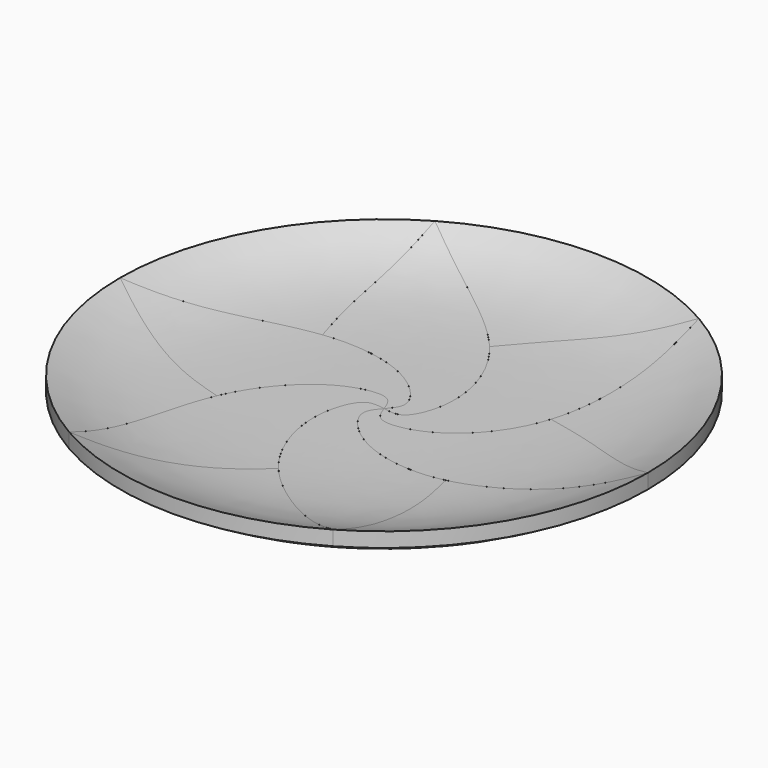
from build123d import *

# Parameters (mm, degrees)
F1_DEPTH  = 25.4
F2_ANGLE  = 60
F3_ANGLE  = 60
F4_ANGLE  = 180
F6_DEPTH  = 25.4
F10_R     = 127
F11_DEPTH = 25.4


# Not quite as in the source:
# - after a boolean that leaves OpenCascade's solid faulty, fix() repairs it


with BuildPart() as f1:
    # F0 (on Top) → F1 (new body)
    with BuildSketch(Plane.XY):
        with BuildLine():
            add(Edge.make_bspline(
                [(57.15, 98.9867036526), (42.865067123, 90.4469959657), (18.1027123706, 75.6437572636), (5.3822632476, 62.6485279549), (0, 57.15)],
                knots=[0, 0, 0, 0, 0.5768810366, 1, 1, 1, 1], degree=3))
            add(Edge.make_bspline(
                [(0, 57.15), (8.9985258992, 46.3479694325), (16.2629547968, 26.203873404), (13.5159669265, 7.6914102768), (7.916444084, -1.4444323794), (2.5428274827, -0.4639636574), (0, 0)],
                knots=[0.3474335303, 0.3474335303, 0.3474335303, 0.3474335303, 0.5931061356, 0.7668229008, 0.8896592034, 1, 1, 1, 1], degree=3))
            add(Edge.make_bspline(
                [(57.15, 98.9867036526), (56.7550823402, 73.1103955813), (56.0809157252, 28.9367746008), (30.8246974438, -0.9821952926), (13.4189401539, -7.8594655767), (2.7073069074, -7.578057874), (0.8696094276, -2.4341350262), (0, 0)],
                knots=[0, 0, 0, 0, 0.3474335303, 0.5931061356, 0.7668229008, 0.8896592034, 1, 1, 1, 1], degree=3))
        make_face()
    extrude(amount=F1_DEPTH)


with BuildPart() as f2_1:
    # F2: copy of F1
    add(f1.part.rotate(Axis((0, 0, 12.7), (0, 0, -1)), F2_ANGLE))


with BuildPart() as f3_1:
    # F3: copy of F2_1
    add(f2_1.part.rotate(Axis((0, 0, 12.7), (0, 0, -1)), F3_ANGLE))


with BuildPart() as f4_1:
    # F4: copy of F3_1
    add(f3_1.part.rotate(Axis((0, 0, 12.7), (0, 0, -1)), F4_ANGLE))


with BuildPart() as f4_2:
    # F4: copy of F2_1
    add(f2_1.part.rotate(Axis((0, 0, 12.7), (0, 0, -1)), F4_ANGLE))


with BuildPart() as f4_3:
    # F4: copy of F1
    add(f1.part.rotate(Axis((0, 0, 12.7), (0, 0, -1)), F4_ANGLE))


with BuildPart() as f6:
    # F5 (on face) → F6 (new body)
    with BuildSketch(Plane.XY.offset(25.4)):
        with BuildLine():
            ThreePointArc((-57.15, 98.9867036526), (-57.15, -98.9867036526), (114.3, 0))
            ThreePointArc((114.3, 0), (57.15, 98.9867036526), (-57.15, 98.9867036526))
        make_face()
        with BuildLine():
            add(Edge.make_bspline(
                [(-57.15, 98.9867036526), (-56.8968626408, 82.3457350463), (-56.4580592426, 53.4992874222), (-51.5640850948, 35.9854406797), (-49.4933518263, 28.575)],
                knots=[0, 0, 0, 0, 0.5768810366, 1, 1, 1, 1], degree=3))
            add(Edge.make_bspline(
                [(-57.15, 98.9867036526), (-34.937918684, 85.7065408912), (2.9804759547, 63.0358849859), (16.2629547968, 26.203873404), (13.5159669265, 7.6914102768), (7.916444084, -1.4444323794), (2.5428274827, -0.4639636574), (0, 0)],
                knots=[0, 0, 0, 0, 0.3474335303, 0.5931061356, 0.7668229008, 0.8896592034, 1, 1, 1, 1], degree=3))
            add(Edge.make_bspline(
                [(-49.4933518263, 28.575), (-35.6392559927, 30.9669367416), (-14.561742647, 27.1860686966), (0.0970267726, 15.5508758535), (5.2091371766, 6.1336254947), (1.6732180551, 1.9701713687), (0, 0)],
                knots=[0.3474335303, 0.3474335303, 0.3474335303, 0.3474335303, 0.5931061356, 0.7668229008, 0.8896592034, 1, 1, 1, 1], degree=3))
        make_face(mode=Mode.SUBTRACT)
    extrude(amount=-F6_DEPTH)

    # F7: cut F2_1, F4_2, F3_1, F4_3, F4_1, F1
    add(f2_1.part, mode=Mode.SUBTRACT)
    add(f4_2.part, mode=Mode.SUBTRACT)
    add(f3_1.part, mode=Mode.SUBTRACT)
    add(f4_3.part, mode=Mode.SUBTRACT)
    add(f4_1.part, mode=Mode.SUBTRACT)
    add(f1.part, mode=Mode.SUBTRACT)


with BuildPart() as f9:
    # F8 (on Front) → F9 (revolve)
    with BuildSketch(Plane.XZ):
        with BuildLine():
            Line((-25.4, 0), (0, 0))
            Line((0, 0), (0, 12.7))
            add(Edge.make_bspline(
                [(-114.3, 25.4), (-101.7942801118, 19.8076143861), (-77.7917917732, 11.5946885383), (-25.5843241359, 12.7), (0, 12.7)],
                knots=[0, 0, 0, 0, 0.4152344317, 1, 1, 1, 1], degree=3))
            Line((-114.3, 25.4), (-114.3, 19.05))
            add(Edge.make_bspline(
                [(-114.3, 19.05), (-104.6237623196, 12.7), (-79.3372868945, 6.4163393889), (-45.5824566747, 5.0293225141), (-24.5591314222, 3.6541606008)],
                knots=[0, 0, 0, 0, 0.4427035027, 1, 1, 1, 1], degree=3))
            Line((-24.5591314222, 3.6541606008), (-25.4, 0))
        make_face()
    revolve(axis=Axis((0, 0, 6.35), (0, 0, 1)))


with BuildPart() as f11:
    # F10 (on Top) → F11 (new body)
    with BuildSketch(Plane.XY):
        Circle(F10_R)
    extrude(amount=F11_DEPTH)

    # F12: cut F9
    add(f9.part, mode=Mode.SUBTRACT)


with BuildPart() as f6_1:
    add(f6.part)

    # F13: cut F11
    add(f11.part, mode=Mode.SUBTRACT)


with BuildPart() as f1_1:
    add(f1.part)

    # F13: cut F11
    add(f11.part, mode=Mode.SUBTRACT)


with BuildPart() as f2_1_1:
    add(f2_1.part)

    # F13: cut F11
    add(f11.part, mode=Mode.SUBTRACT)


with BuildPart() as f3_1_1:
    add(f3_1.part)

    # F13: cut F11
    add(f11.part, mode=Mode.SUBTRACT)


with BuildPart() as f4_3_1:
    add(f4_3.part)

    # F13: cut F11
    add(f11.part, mode=Mode.SUBTRACT)

    add(f4_3_1.part.fix(), mode=Mode.REPLACE)


with BuildPart() as f4_2_1:
    add(f4_2.part)

    # F13: cut F11
    add(f11.part, mode=Mode.SUBTRACT)

    add(f4_2_1.part.fix(), mode=Mode.REPLACE)


with BuildPart() as f4_1_1:
    add(f4_1.part)

    # F13: cut F11
    add(f11.part, mode=Mode.SUBTRACT)


solid = Compound([f6_1.part, f1_1.part, f2_1_1.part, f3_1_1.part, f4_3_1.part, f4_2_1.part, f4_1_1.part])
